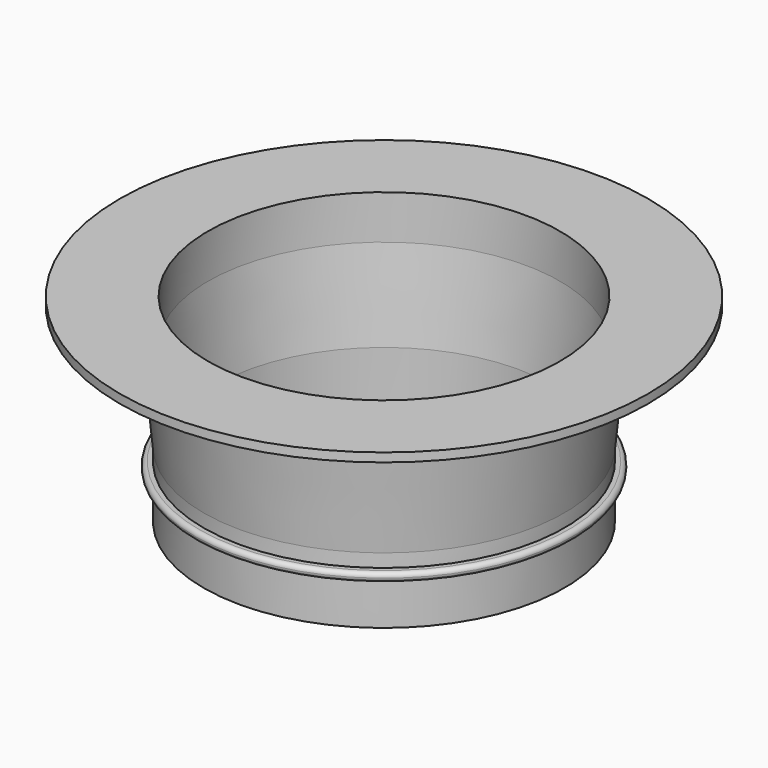
from build123d import *

# Parameters (mm, degrees)
F2_R     = 76.2
F2_R_2   = 54.6292916326
F2_R_3   = 52.1095022643
F3_DEPTH = 2.54
F4_R     = 1.26999


# Not quite as in the source:
# - a fillet or chamfer is up to 0.001 mm smaller than in the source, because OpenCascade refuses the exact size


with BuildPart() as f1:
    # F0 (on Right) → F1 (revolve)
    with BuildSketch(Plane.YZ):
        Polygon((-48.2407083674, -19.05), (-48.2407083674, 0), (-50.8, 25.4), (-50.8, 38.1), (-54.6292916326, 38.1), (-54.6292916326, 25.4), (-52.07, 0), (-52.07, -3.81), (-54.61, -3.81), (-54.61, -6.35), (-52.07, -6.35), (-52.07, -19.05), align=None)
    revolve(axis=Axis((0, 0, 19.0012101084), (0, 0, -1)))

    # F2 (on face) → F3 (join)
    with BuildSketch(Plane.XY.offset(38.1)):
        Circle(F2_R)
        Circle(F2_R_2, mode=Mode.SUBTRACT)
        Circle(F2_R_2)
        Circle(F2_R_3, mode=Mode.SUBTRACT)
    extrude(amount=-F3_DEPTH)

    # F4 (radius 1.27 in the source; OpenCascade refuses exactly that, so slightly less here)
    f4_edges = [f1.edges().sort_by_distance(p)[0] for p in [
        (0, 54.61, -3.81),
        (0, 54.61, -6.35),
    ]]
    fillet(f4_edges, radius=F4_R)


solid = f1.part
